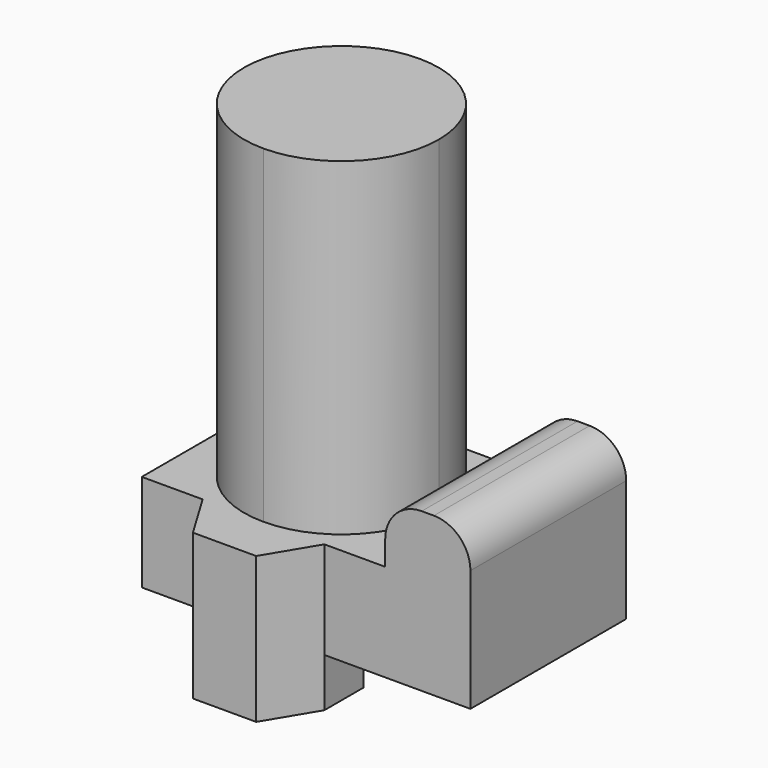
from build123d import *

# Parameters (mm, degrees)
F1_DEPTH = 80
F3_DEPTH = 135
F5_DEPTH = 60
F6_R     = 3
F7_DEPTH = 10


# Not quite as in the source:
# - a feature names something its author has since deleted; it is built from what else it names


with BuildPart() as f1:
    # F0 (on Front) → F1 (new body)
    with BuildSketch(Plane.XZ):
        with BuildLine():
            Line((-135, 0), (0, 0))
            Line((0, 0), (0, 50))
            ThreePointArc((0, 50), (-4.3933982822, 60.6066017178), (-15, 65))
            Line((-15, 65), (-20, 65))
            ThreePointArc((-20, 65), (-30.6066017178, 60.6066017178), (-35, 50))
            Line((-35, 50), (-35, 40))
            Line((-35, 40), (-135, 40))
            Line((-135, 40), (-135, 0))
        make_face()
    extrude(amount=F1_DEPTH)

    # F2 (on face) → F3 (join)
    with BuildSketch(Plane.XY.offset(40)):
        with BuildLine():
            ThreePointArc((-45, -40), (-56.7157287525, -11.7157287525), (-85, 0))
            ThreePointArc((-85, 0), (-125, -40), (-85, -80))
            ThreePointArc((-85, -80), (-56.7157287525, -68.2842712475), (-45, -40))
        make_face()
    extrude(amount=F3_DEPTH)

    # F4 (on face) → F5 (join)
    with BuildSketch(Plane.XY.offset(40)):
        with BuildLine():
            Line((-60, -60), (-110, -60))
            Line((-110, -60), (-110, -71.224989992))
            ThreePointArc((-110, -71.224989992), (-98.247648854, -77.7425462819), (-85, -80))
            ThreePointArc((-85, -80), (-71.7523511459, -77.7425462819), (-60, -71.224989992))
            Line((-60, -71.224989992), (-60, -60))
        make_face()
        with BuildLine():
            ThreePointArc((-85, -80), (-98.247648854, -77.7425462819), (-110, -71.224989992))
            Line((-110, -71.224989992), (-110, -80))
            Line((-110, -80), (-98, -100))
            Line((-98, -100), (-72, -100))
            Line((-72, -100), (-60, -80))
            Line((-60, -80), (-85, -80))
        make_face()
        with BuildLine():
            Line((-60, -80), (-60, -71.224989992))
            ThreePointArc((-60, -71.224989992), (-71.7523511459, -77.7425462819), (-85, -80))
            Line((-85, -80), (-60, -80))
        make_face()
    extrude(amount=-F5_DEPTH)

    # F6 (on face) → F7 (cut)
    with BuildSketch(Plane(origin=(0, 0, 0), x_dir=(-1, 0, 0), z_dir=(0, 1, 0))):
        with Locations((65, 20)):
            Circle(F6_R)
    extrude(amount=-F7_DEPTH, mode=Mode.SUBTRACT)


solid = f1.part
